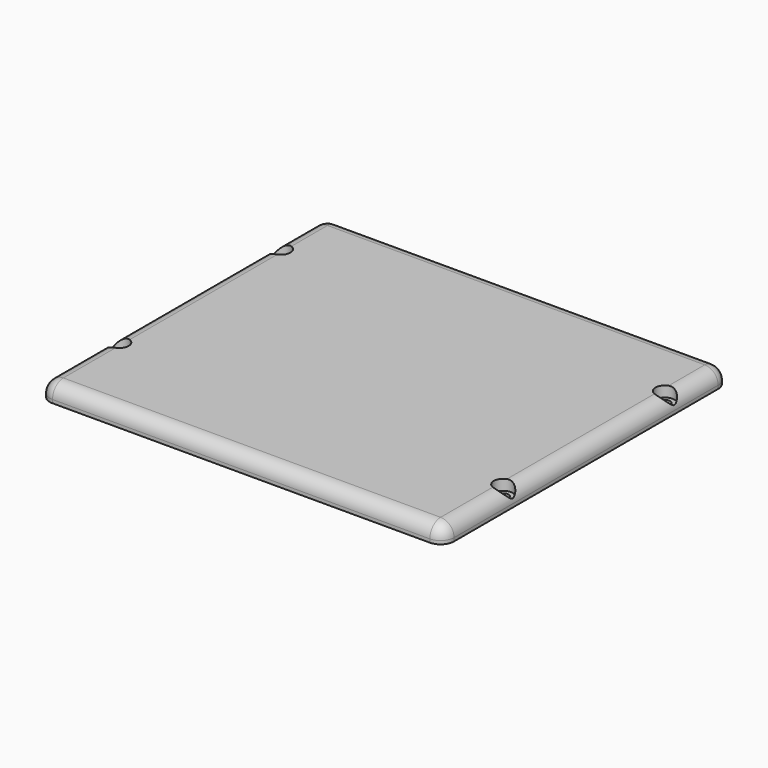
from build123d import *

# Parameters (mm, degrees)
F0_W           = 152.4
F0_H           = 134.62
F1_DEPTH       = 6.35
F3_D           = 3.9878
F3_CBORE_D     = 7.112
F3_CBORE_DEPTH = 4.000000001
F4_T1_DEPTH    = 124.46
F4_T3_DEPTH    = 142.24
F4_T5_DEPTH    = 13.97
F4_S9_W        = 5.08
F4_S9_H        = 5.08
F4_T10_DEPTH   = 5.08
F4_S15_W       = 5.08
F4_S15_H       = 5.08
F4_T16_DEPTH   = 5.08
F4_S21_W       = 5.08
F4_S21_H       = 5.08
F4_T22_DEPTH   = 5.08
F4_S27_W       = 5.08
F4_S27_H       = 5.08
F4_T28_DEPTH   = 5.08


# Not quite as in the source:
# - a fillet or chamfer that OpenCascade refuses, or shapes differently, is made with other operations: its cross-section is extruded or revolved along the edge and cut away or added
# - a feature names something its author has since deleted; it is built from what else it names


with BuildPart() as f1:
    # F0 (on Top) → F1 (new body)
    with BuildSketch(Plane.XY):
        Rectangle(F0_W, F0_H)
    extrude(amount=F1_DEPTH)

    # F3 (through all)
    with Locations(Plane.XY.offset(6.35)):
        with Locations((-72.39, 41.91), (-72.39, -34.29), (72.39, -34.29), (72.39, 41.91)):
            CounterBoreHole(F3_D / 2, F3_CBORE_D / 2, F3_CBORE_DEPTH)

    # F4: fillet of radius 5.08 on 8 edges, made by hand

    # F4_s2 → F4_t1 (cut)
    with BuildSketch(Plane.XZ.offset(-62.23)):
        with BuildLine():
            ThreePointArc((-76.2, 1.27), (-74.7121024484, 4.8621024484), (-71.12, 6.35))
            Line((-71.12, 6.35), (-76.2, 6.35))
            Line((-76.2, 6.35), (-76.2, 1.27))
        make_face()
        with BuildLine():
            ThreePointArc((76.2, 1.27), (74.7121024484, 4.8621024484), (71.12, 6.35))
            Line((71.12, 6.35), (76.2, 6.35))
            Line((76.2, 6.35), (76.2, 1.27))
        make_face()
    extrude(amount=F4_T1_DEPTH, mode=Mode.SUBTRACT)

    # F4_s4 → F4_t3 (cut)
    with BuildSketch(Plane.YZ.offset(-71.12)):
        with BuildLine():
            ThreePointArc((62.23, 6.35), (65.8221024484, 4.8621024484), (67.31, 1.27))
            Line((67.31, 1.27), (67.31, 6.35))
            Line((67.31, 6.35), (62.23, 6.35))
        make_face()
        with BuildLine():
            ThreePointArc((-67.31, 1.27), (-65.8221024484, 4.8621024484), (-62.23, 6.35))
            Line((-62.23, 6.35), (-67.31, 6.35))
            Line((-67.31, 6.35), (-67.31, 1.27))
        make_face()
    extrude(amount=F4_T3_DEPTH, mode=Mode.SUBTRACT)

    # F4_s6 → F4_t5 (cut)
    with BuildSketch(Plane.XY.offset(-12.7)):
        with BuildLine():
            ThreePointArc((-71.12, -67.31), (-74.7121024484, -65.8221024484), (-76.2, -62.23))
            Line((-76.2, -62.23), (-76.2, -67.31))
            Line((-76.2, -67.31), (-71.12, -67.31))
        make_face()
        with BuildLine():
            ThreePointArc((71.12, -67.31), (74.7121024484, -65.8221024484), (76.2, -62.23))
            Line((76.2, -62.23), (76.2, -67.31))
            Line((76.2, -67.31), (71.12, -67.31))
        make_face()
        with BuildLine():
            ThreePointArc((76.2, 62.23), (74.7121024484, 65.8221024484), (71.12, 67.31))
            Line((71.12, 67.31), (76.2, 67.31))
            Line((76.2, 67.31), (76.2, 62.23))
        make_face()
        with BuildLine():
            ThreePointArc((-76.2, 62.23), (-74.7121024484, 65.8221024484), (-71.12, 67.31))
            Line((-71.12, 67.31), (-76.2, 67.31))
            Line((-76.2, 67.31), (-76.2, 62.23))
        make_face()
    extrude(amount=F4_T5_DEPTH, mode=Mode.SUBTRACT)


with BuildPart() as f4_tool8:
    # F4_s9 → F4_t10 (new body)
    with BuildSketch(Plane.YZ.offset(-71.12)):
        with Locations((64.77, 3.81)):
            Rectangle(F4_S9_W, F4_S9_H)
    extrude(amount=-F4_T10_DEPTH)

    # F4_s11 → F4_t12 (revolve, cut)
    with BuildSketch(Plane(origin=(-71.12, 62.23, 1.27), x_dir=(0, -0.7071067812, -0.7071067812), z_dir=(0, 0.7071067812, -0.7071067812))):
        with BuildLine():
            ThreePointArc((0, -5.08), (5.08, 0), (0, 5.08))
            Line((0, 5.08), (0, -5.08))
        make_face()
    revolve(axis=Axis((-71.12, 62.23, 1.27), (-1, 0, 0)), mode=Mode.SUBTRACT)


with BuildPart() as f1_1:
    add(f1.part)

    # F4_t7: cut F4_tool8
    add(f4_tool8.part, mode=Mode.SUBTRACT)


with BuildPart() as f4_tool14:
    # F4_s15 → F4_t16 (new body)
    with BuildSketch(Plane.XZ.offset(62.23)):
        with Locations((-73.66, 3.81)):
            Rectangle(F4_S15_W, F4_S15_H)
    extrude(amount=F4_T16_DEPTH)

    # F4_s17 → F4_t18 (revolve, cut)
    with BuildSketch(Plane(origin=(-71.12, -62.23, 1.27), x_dir=(0.7071067812, 0, -0.7071067812), z_dir=(-0.7071067812, 0, -0.7071067812))):
        with BuildLine():
            ThreePointArc((0, -5.08), (5.08, 0), (0, 5.08))
            Line((0, 5.08), (0, -5.08))
        make_face()
    revolve(axis=Axis((-71.12, -62.23, 1.27), (0, -1, 0)), mode=Mode.SUBTRACT)


with BuildPart() as f1_2:
    add(f1_1.part)

    # F4_t13: cut F4_tool14
    add(f4_tool14.part, mode=Mode.SUBTRACT)


with BuildPart() as f4_tool20:
    # F4_s21 → F4_t22 (new body)
    with BuildSketch(Plane.YZ.offset(71.12)):
        with Locations((64.77, 3.81)):
            Rectangle(F4_S21_W, F4_S21_H)
    extrude(amount=F4_T22_DEPTH)

    # F4_s23 → F4_t24 (revolve, cut)
    with BuildSketch(Plane(origin=(71.12, 62.23, 1.27), x_dir=(0, -0.7071067812, -0.7071067812), z_dir=(0, -0.7071067812, 0.7071067812))):
        with BuildLine():
            ThreePointArc((0, -5.08), (5.08, 0), (0, 5.08))
            Line((0, 5.08), (0, -5.08))
        make_face()
    revolve(axis=Axis((71.12, 62.23, 1.27), (1, 0, 0)), mode=Mode.SUBTRACT)


with BuildPart() as f1_3:
    add(f1_2.part)

    # F4_t19: cut F4_tool20
    add(f4_tool20.part, mode=Mode.SUBTRACT)


with BuildPart() as f4_tool26:
    # F4_s27 → F4_t28 (new body)
    with BuildSketch(Plane.XZ.offset(62.23)):
        with Locations((73.66, 3.81)):
            Rectangle(F4_S27_W, F4_S27_H)
    extrude(amount=F4_T28_DEPTH)

    # F4_s29 → F4_t30 (revolve, cut)
    with BuildSketch(Plane(origin=(71.12, -62.23, 1.27), x_dir=(-0.7071067812, 0, -0.7071067812), z_dir=(-0.7071067812, 0, 0.7071067812))):
        with BuildLine():
            ThreePointArc((0, -5.08), (5.08, 0), (0, 5.08))
            Line((0, 5.08), (0, -5.08))
        make_face()
    revolve(axis=Axis((71.12, -62.23, 1.27), (0, -1, 0)), mode=Mode.SUBTRACT)


with BuildPart() as f1_4:
    add(f1_3.part)

    # F4_t25: cut F4_tool26
    add(f4_tool26.part, mode=Mode.SUBTRACT)


solid = f1_4.part
